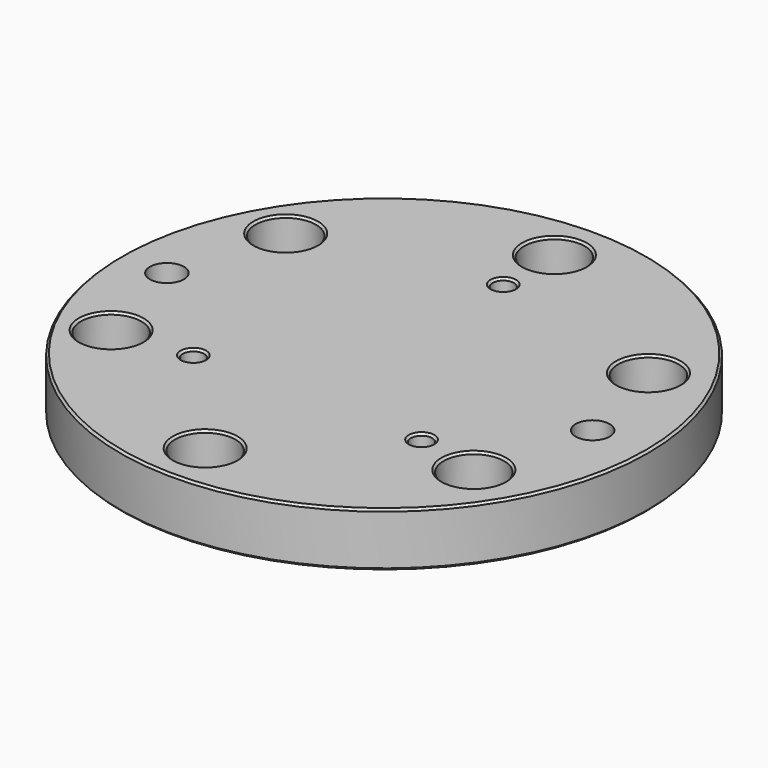
from build123d import *

# Parameters (mm, degrees)
F0_R           = 62
F1_DEPTH       = 12.7
F2_D           = 5
F4_D           = 9
F4_CBORE_D     = 14.25
F4_CBORE_DEPTH = 8
F5_SIZE        = 0.5
F6_D           = 8


# Not quite as in the source:
# - a feature names something its author has since deleted; it is built from what else it names


with BuildPart() as f1:
    # F0 (on Top) → F1 (new body)
    with BuildSketch(Plane.XY):
        Circle(F0_R)
    extrude(amount=F1_DEPTH)

    # F2 (through all)
    with Locations(Plane(origin=(0, 0, 0), x_dir=(1, 0, 0), z_dir=(0, 0, -1))):
        with Locations((0, -35), (26.8, 22.5), (-26.8, 22.5)):
            Hole(F2_D / 2)

    # F4 (through all)
    with Locations(Plane.XY.offset(12.7)):
        with Locations((0, 50), (-43.8068557852, 25.8756999398), (42.7956845933, 24.1243000602), (-44.8180269771, -24.1243000602), (-2.0223423839, -50), (41.7845134013, -25.8756999398)):
            CounterBoreHole(F4_D / 2, F4_CBORE_D / 2, F4_CBORE_DEPTH)

    # F5
    f5_edges = [f1.edges().sort_by_distance(p)[0] for p in [
        (-62, 0, 12.7),
        (-9.147342, -50, 12.7),
        (-51.943027, -24.1243, 12.7),
        (-29.3, -22.5, 12.7),
        (24.3, -22.5, 12.7),
        (34.659513, -25.8757, 12.7),
        (-50.931856, 25.8757, 12.7),
        (35.670685, 24.1243, 12.7),
        (-2.5, 35, 12.7),
        (-7.125, 50, 12.7),
        (-62, 0, 0),
        (-6.522342, -50, 0),
        (-49.318027, -24.1243, 0),
        (-29.3, -22.5, 0),
        (24.3, -22.5, 0),
        (37.284513, -25.8757, 0),
        (-48.306856, 25.8757, 0),
        (38.295685, 24.1243, 0),
        (-2.5, 35, 0),
        (-4.5, 50, 0),
    ]]
    chamfer(f5_edges, length=F5_SIZE)

    # F6 (through all)
    with Locations(Plane.XY.offset(12.7)):
        with Locations((-51.0111711919, 0), (48.9888288081, 0)):
            Hole(F6_D / 2)


solid = f1.part
